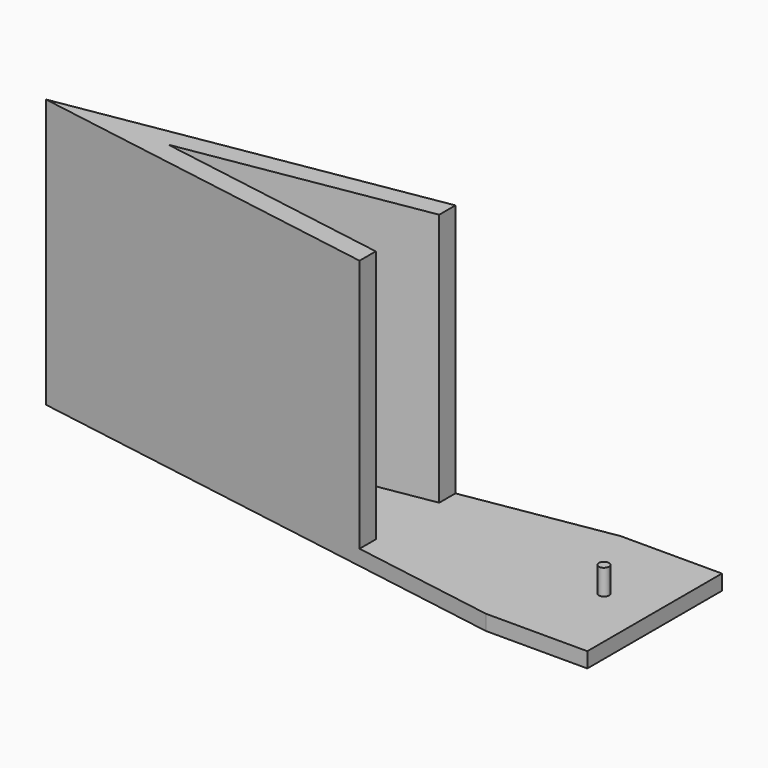
from build123d import *

# Parameters (mm, degrees)
F1_DEPTH = 1.5
F3_DEPTH = 25
F4_R     = 0.5
F5_DEPTH = 2.5


# Not quite as in the source:
# - a feature names something its author has since deleted; it is built from what else it names


with BuildPart() as f1:
    # F0 (on Top) → F1 (new body)
    with BuildSketch(Plane.XY):
        Polygon((-37.5444034434, -27.2088618949), (12.4555965566, -35.5019792914), (22.4555965566, -35.5019792914), (22.4555965566, -18.9157444984), (12.4555965566, -18.9157444984), align=None)
    extrude(amount=F1_DEPTH)

    # F2 (on face) → F3 (join)
    with BuildSketch(Plane.XY.offset(1.5)):
        Polygon((-37.5444034434, -27.2088618949), (-1.9112733802, -33.1190565113), (-1.9112733802, -31.1190565113), (-25.486211666, -27.2088618949), (-1.9112733802, -23.2986672785), (-1.9112733802, -21.2986672785), align=None)
    extrude(amount=F3_DEPTH)

    # F4 (on face) → F5 (join)
    with BuildSketch(Plane.XY.offset(1.5)):
        with Locations((17.4555965566, -27.2088618949)):
            Circle(F4_R)
    extrude(amount=F5_DEPTH)


solid = f1.part
